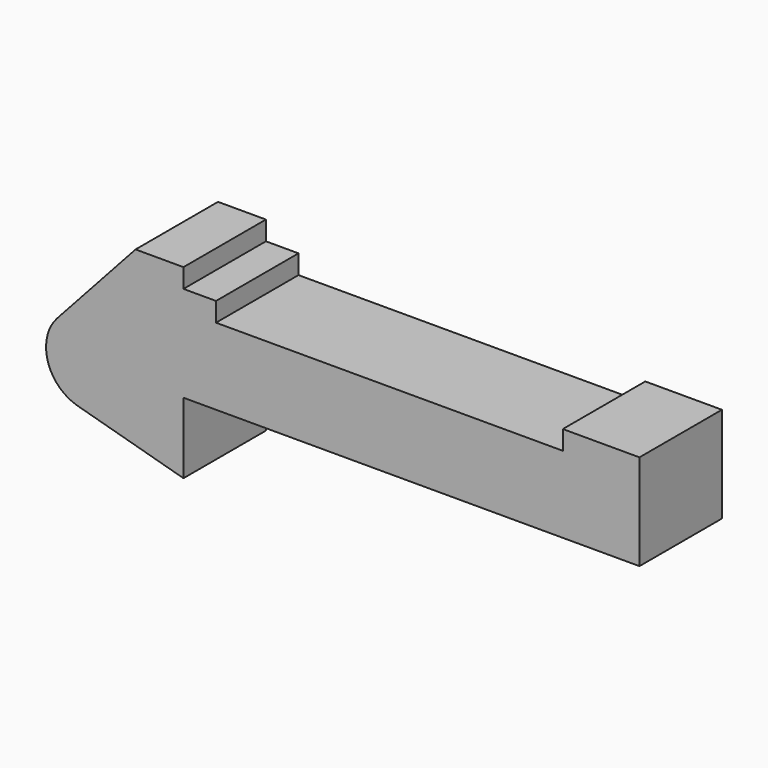
from build123d import *

# Parameters (mm, degrees)
F0_R     = 3.175
F0_W     = 5.842
F0_H     = 12.7
F1_DEPTH = 13.6652


with BuildPart() as f1:
    # F0 (on Front) → F1 (new body)
    with BuildSketch(Plane.XZ):
        Polygon((5.842, 12.7), (5.842, 0), (66.294, 0), (66.294, 12.7), (56.134, 12.7), (56.134, 10.16), (10.16, 10.16), (10.16, 12.7), align=None)
        with BuildLine():
            ThreePointArc((-8.1826630726, -5.5069827884), (-3.1957909266, -4.5493385486), (-0.9398, 0))
            ThreePointArc((-0.9398, 0), (-4.5919612295, 5.3297205562), (-10.8806298187, 3.8475430269))
            ThreePointArc((-10.8806298187, 3.8475430269), (-12.1459778134, -1.5837270034), (-8.1826630726, -5.5069827884))
        make_face()
        with Locations((-6.6548, 0)):
            Circle(F0_R, mode=Mode.SUBTRACT)
        with BuildLine():
            Line((-0.9398, 0), (0, 0))
            Line((0, 0), (0, 12.7))
            Line((0, 12.7), (5.842, 12.7))
            Line((5.842, 12.7), (5.842, 15.24))
            Line((5.842, 15.24), (-0.508, 15.24))
            Line((-0.508, 15.24), (-10.8806298187, 3.8475430269))
            ThreePointArc((-10.8806298187, 3.8475430269), (-4.5919612295, 5.3297205562), (-0.9398, 0))
        make_face()
        with Locations((2.921, 6.35)):
            Rectangle(F0_W, F0_H)
        with BuildLine():
            Line((5.842, 0), (0, 0))
            Line((0, 0), (-0.9398, 0))
            ThreePointArc((-0.9398, 0), (-3.1957909266, -4.5493385486), (-8.1826630726, -5.5069827884))
            Line((-8.1826630726, -5.5069827884), (5.842, -9.398))
            Line((5.842, -9.398), (5.842, 0))
        make_face()
        with Locations((-6.6548, 0)):
            Circle(F0_R)
    extrude(amount=F1_DEPTH)


solid = f1.part
